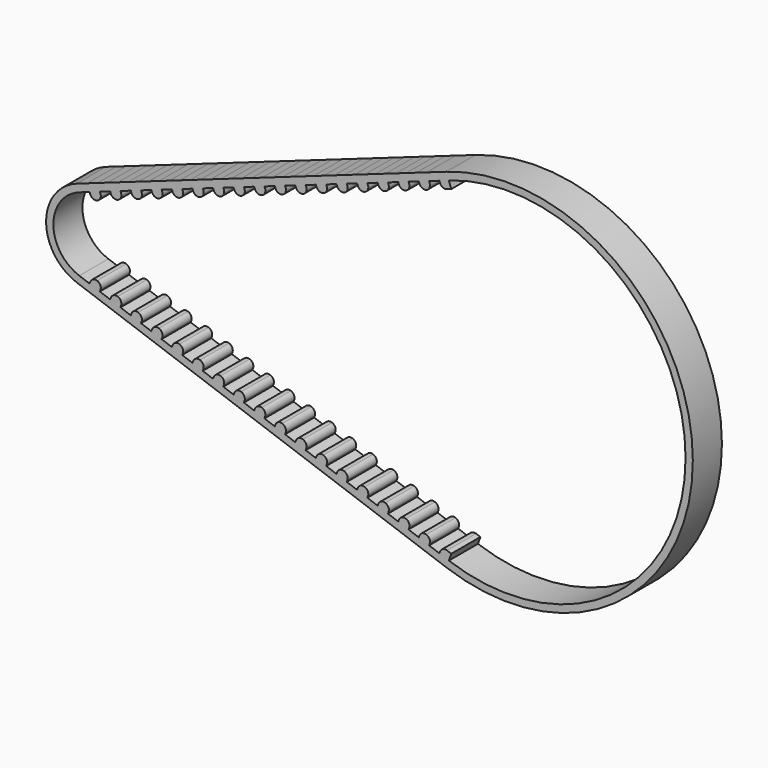
from build123d import *

# Parameters (mm, degrees)
F1_DEPTH = 10
F2_T     = -2
F3_W     = 3
F3_H     = 10
F3_W_2   = 2.7630734528
F4_DEPTH = 4
F5_R     = 1.5
F6_R     = 1.49999
F7_W     = 3
F7_H     = 10
F7_W_2   = 2.7630734528
F8_DEPTH = 4
F9_R     = 1.49999


# Not quite as in the source:
# - a fillet or chamfer is up to 0.001 mm smaller than in the source, because OpenCascade refuses the exact size


with BuildPart() as f1:
    # F0 (on Front) → F1 (new body)
    with BuildSketch(Plane.XZ):
        with BuildLine():
            Line((21.5677155773, 47.8946993124), (-80.0322844227, 11.9736748281))
            ThreePointArc((-80.0322844227, 11.9736748281), (-88.4989510894, 0), (-80.0322844227, -11.9736748281))
            Line((-80.0322844227, -11.9736748281), (21.5677155773, -47.8946993124))
            ThreePointArc((21.5677155773, -47.8946993124), (89.3010489106, 0), (21.5677155773, 47.8946993124))
        make_face()
    extrude(amount=F1_DEPTH)

    # F2
    f2_openings = [f1.faces().sort_by_distance(p)[0] for p in [
        (13.860762, -10, 0),
        (13.860762, 0, 0),
    ]]
    offset(amount=F2_T, openings=f2_openings)

    # F3 (on face) → F4 (join)
    with BuildSketch(Plane(origin=(-12.6554390099, 0, 35.7949869713), x_dir=(0.9428090416, 0, 0.3333333333), z_dir=(-0.3333333333, 0, 0.9428090416))):
        with Locations((-66.9639364295, -5)):
            Rectangle(F3_W, F3_H)
        with Locations((-60.9639364295, -5)):
            Rectangle(F3_W, F3_H)
        with Locations((-54.9639364295, -5)):
            Rectangle(F3_W, F3_H)
        with Locations((-48.9639364295, -5)):
            Rectangle(F3_W, F3_H)
        with Locations((-42.9639364295, -5)):
            Rectangle(F3_W, F3_H)
        with Locations((-36.9639364295, -5)):
            Rectangle(F3_W, F3_H)
        with Locations((-30.9639364295, -5)):
            Rectangle(F3_W, F3_H)
        with Locations((-24.9639364295, -5)):
            Rectangle(F3_W, F3_H)
        with Locations((-18.9639364295, -5)):
            Rectangle(F3_W, F3_H)
        with Locations((-12.9639364295, -5)):
            Rectangle(F3_W, F3_H)
        with Locations((-6.9639364295, -5)):
            Rectangle(F3_W, F3_H)
        with Locations((-0.9639364295, -5)):
            Rectangle(F3_W, F3_H)
        with Locations((5.0360635705, -5)):
            Rectangle(F3_W, F3_H)
        with Locations((11.0360635705, -5)):
            Rectangle(F3_W, F3_H)
        with Locations((17.0360635705, -5)):
            Rectangle(F3_W, F3_H)
        with Locations((23.0360635705, -5)):
            Rectangle(F3_W, F3_H)
        with Locations((29.0360635705, -5)):
            Rectangle(F3_W, F3_H)
        with Locations((34.9176002969, -5)):
            Rectangle(F3_W_2, F3_H)
    extrude(amount=-F4_DEPTH)

    # F5
    f5_edges = [f1.edges().sort_by_distance(p)[0] for p in [
        (-75.870524, -5, 9.202439),
    ]]
    fillet(f5_edges, radius=F5_R)

    # F6 (radius 1.5 in the source; OpenCascade refuses exactly that, so slightly less here)
    f6_edges = [f1.edges().sort_by_distance(p)[0] for p in [
        (-73.042097, -5, 10.202439),
        (-70.21367, -5, 11.202439),
        (-67.385243, -5, 12.202439),
        (-64.556815, -5, 13.202439),
        (-61.728388, -5, 14.202439),
        (-58.899961, -5, 15.202439),
        (-56.071534, -5, 16.202439),
        (-53.243107, -5, 17.202439),
        (-50.41468, -5, 18.202439),
        (-47.586253, -5, 19.202439),
        (-44.757826, -5, 20.202439),
        (-41.929398, -5, 21.202439),
        (-39.100971, -5, 22.202439),
        (-36.272544, -5, 23.202439),
        (-33.444117, -5, 24.202439),
        (-30.61569, -5, 25.202439),
        (-27.787263, -5, 26.202439),
        (-24.958836, -5, 27.202439),
        (-22.130409, -5, 28.202439),
        (-19.301981, -5, 29.202439),
        (-16.473554, -5, 30.202439),
        (-13.645127, -5, 31.202439),
        (-10.8167, -5, 32.202439),
        (-7.988273, -5, 33.202439),
        (-5.159846, -5, 34.202439),
        (-2.331419, -5, 35.202439),
        (0.497008, -5, 36.202439),
        (3.325436, -5, 37.202439),
        (6.153863, -5, 38.202439),
        (8.98229, -5, 39.202439),
        (11.810717, -5, 40.202439),
        (14.639144, -5, 41.202439),
        (17.467571, -5, 42.202439),
        (20.295998, -5, 43.202439),
    ]]
    fillet(f6_edges, radius=F6_R)

    # F7 (on face) → F8 (join)
    with BuildSketch(Plane(origin=(-12.6554390099, 0, -35.7949869713), x_dir=(0.9428090416, 0, -0.3333333333), z_dir=(-0.3333333333, 0, -0.9428090416))):
        with Locations((-66.9639364295, 5)):
            Rectangle(F7_W, F7_H)
        with Locations((-60.9639364295, 5)):
            Rectangle(F7_W, F7_H)
        with Locations((-54.9639364295, 5)):
            Rectangle(F7_W, F7_H)
        with Locations((-48.9639364295, 5)):
            Rectangle(F7_W, F7_H)
        with Locations((-42.9639364295, 5)):
            Rectangle(F7_W, F7_H)
        with Locations((-36.9639364295, 5)):
            Rectangle(F7_W, F7_H)
        with Locations((-30.9639364295, 5)):
            Rectangle(F7_W, F7_H)
        with Locations((-24.9639364295, 5)):
            Rectangle(F7_W, F7_H)
        with Locations((-18.9639364295, 5)):
            Rectangle(F7_W, F7_H)
        with Locations((-12.9639364295, 5)):
            Rectangle(F7_W, F7_H)
        with Locations((-6.9639364295, 5)):
            Rectangle(F7_W, F7_H)
        with Locations((-0.9639364295, 5)):
            Rectangle(F7_W, F7_H)
        with Locations((5.0360635705, 5)):
            Rectangle(F7_W, F7_H)
        with Locations((11.0360635705, 5)):
            Rectangle(F7_W, F7_H)
        with Locations((17.0360635705, 5)):
            Rectangle(F7_W, F7_H)
        with Locations((23.0360635705, 5)):
            Rectangle(F7_W, F7_H)
        with Locations((29.0360635705, 5)):
            Rectangle(F7_W, F7_H)
        with Locations((34.9176002969, 5)):
            Rectangle(F7_W_2, F7_H)
    extrude(amount=-F8_DEPTH)

    # F9 (radius 1.5 in the source; OpenCascade refuses exactly that, so slightly less here)
    f9_edges = [f1.edges().sort_by_distance(p)[0] for p in [
        (-75.870524, -5, -9.202439),
        (-73.042097, -5, -10.202439),
        (-70.21367, -5, -11.202439),
        (-67.385243, -5, -12.202439),
        (-64.556815, -5, -13.202439),
        (-58.899961, -5, -15.202439),
        (-61.728388, -5, -14.202439),
        (-56.071534, -5, -16.202439),
        (-53.243107, -5, -17.202439),
        (-50.41468, -5, -18.202439),
        (-47.586253, -5, -19.202439),
        (-44.757826, -5, -20.202439),
        (-41.929398, -5, -21.202439),
        (-39.100971, -5, -22.202439),
        (-36.272544, -5, -23.202439),
        (-33.444117, -5, -24.202439),
        (-30.61569, -5, -25.202439),
        (-27.787263, -5, -26.202439),
        (-24.958836, -5, -27.202439),
        (-22.130409, -5, -28.202439),
        (-19.301981, -5, -29.202439),
        (-16.473554, -5, -30.202439),
        (-13.645127, -5, -31.202439),
        (-10.8167, -5, -32.202439),
        (-7.988273, -5, -33.202439),
        (-5.159846, -5, -34.202439),
        (-2.331419, -5, -35.202439),
        (0.497008, -5, -36.202439),
        (3.325436, -5, -37.202439),
        (6.153863, -5, -38.202439),
        (8.98229, -5, -39.202439),
        (11.810717, -5, -40.202439),
        (14.639144, -5, -41.202439),
        (17.467571, -5, -42.202439),
        (20.295998, -5, -43.202439),
    ]]
    fillet(f9_edges, radius=F9_R)


solid = f1.part
